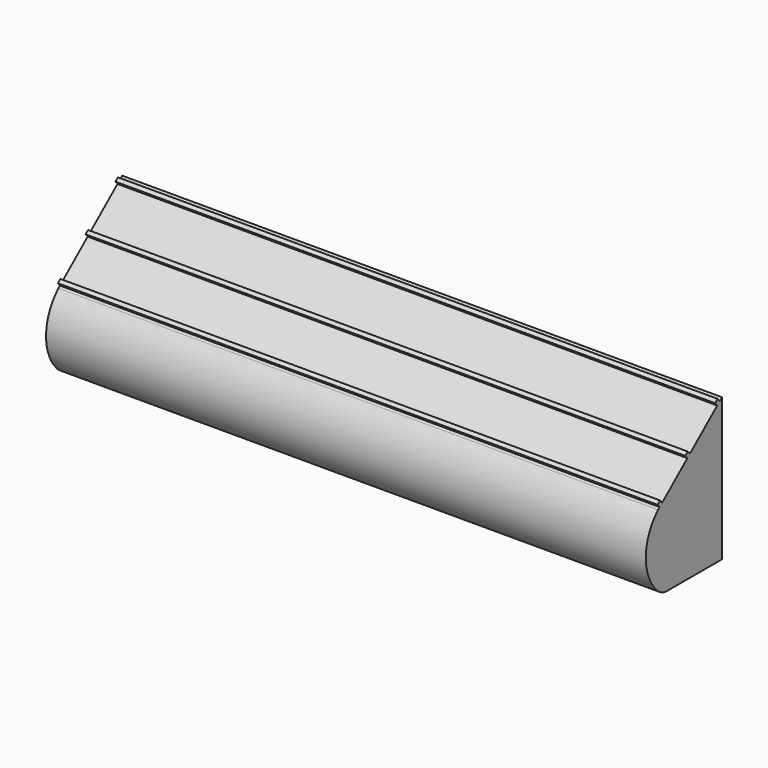
from build123d import *

# Parameters (mm, degrees)
F1_DEPTH    = 55.5
F2_DEPTH    = 297.5
F3_T        = 4
F3_T3_DEPTH = 305.5
F4_R        = 9
F5_R        = 9


# Not quite as in the source:
# - a shell that OpenCascade refuses in one call is made with other operations: the cavity is built on its own and cut out
# - a feature names something its author has since deleted; it is built from what else it names


with BuildPart() as f1:
    # F0 (on Right) → F1 (new body)
    with BuildSketch(Plane.YZ):
        with BuildLine():
            Line((-572.7275457045, -8.2819332473), (-535.7275457045, -8.2819332473))
            Line((-535.7275457045, -8.2819332473), (-535.7275457045, 62.5302098664))
            Line((-535.7275457045, 62.5302098664), (-537.1212494235, 61.363881769))
            Line((-537.1212494235, 61.363881769), (-538.6550321213, 60.0803278606))
            Line((-538.6550321213, 60.0803278606), (-555.619452014, 45.8835661626))
            Line((-555.619452014, 45.8835661626), (-557.1532347119, 44.6000122542))
            Line((-557.1532347119, 44.6000122542), (-572.8000965488, 31.5058557652))
            Line((-572.8000965488, 31.5058557652), (-574.3338792466, 30.2223018568))
            Line((-574.3338792466, 30.2223018568), (-575.2947741996, 29.4181719927))
            ThreePointArc((-575.2947741996, 29.4181719927), (-582.8883712939, 9.9636162879), (-572.7275457045, -8.2819332473))
        make_face()
        Polygon((-538.6550321213, 60.0803278606), (-537.1212494235, 61.363881769), (-538.404803332, 62.8976644668), (-539.9385860298, 61.6141105584), align=None)
        Polygon((-575.6174331551, 31.7560845546), (-574.3338792466, 30.2223018568), (-572.8000965488, 31.5058557652), (-574.0836504573, 33.0396384631), align=None)
        Polygon((-557.1532347119, 44.6000122542), (-555.619452014, 45.8835661626), (-556.9030059225, 47.4173488605), (-558.4367886203, 46.133794952), align=None)
    extrude(amount=F1_DEPTH)

    # F0 (on Right) → F2 (join)
    with BuildSketch(Plane.YZ):
        with BuildLine():
            Line((-572.7275457045, -8.2819332473), (-535.7275457045, -8.2819332473))
            Line((-535.7275457045, -8.2819332473), (-535.7275457045, 62.5302098664))
            Line((-535.7275457045, 62.5302098664), (-537.1212494235, 61.363881769))
            Line((-537.1212494235, 61.363881769), (-538.6550321213, 60.0803278606))
            Line((-538.6550321213, 60.0803278606), (-555.619452014, 45.8835661626))
            Line((-555.619452014, 45.8835661626), (-557.1532347119, 44.6000122542))
            Line((-557.1532347119, 44.6000122542), (-572.8000965488, 31.5058557652))
            Line((-572.8000965488, 31.5058557652), (-574.3338792466, 30.2223018568))
            Line((-574.3338792466, 30.2223018568), (-575.2947741996, 29.4181719927))
            ThreePointArc((-575.2947741996, 29.4181719927), (-582.8883712939, 9.9636162879), (-572.7275457045, -8.2819332473))
        make_face()
        Polygon((-538.6550321213, 60.0803278606), (-537.1212494235, 61.363881769), (-538.404803332, 62.8976644668), (-539.9385860298, 61.6141105584), align=None)
        Polygon((-575.6174331551, 31.7560845546), (-574.3338792466, 30.2223018568), (-572.8000965488, 31.5058557652), (-574.0836504573, 33.0396384631), align=None)
        Polygon((-557.1532347119, 44.6000122542), (-555.619452014, 45.8835661626), (-556.9030059225, 47.4173488605), (-558.4367886203, 46.133794952), align=None)
    extrude(amount=F2_DEPTH)

    # F3: shell of thickness 4, made by hand


with BuildPart() as f3_core1:
    # F3_t2: copy of F1
    add(f1.part)

    # the walls: a layer under each face that stays
    f3_faces = [f3_core1.faces().sort_by_distance(p)[0] for p in [
        (148.75, -582.8883712939, 9.9636162879),
        (0, -559.3362720247, 27.3078656098),
        (148.75, -574.9756562009, 30.9891932057),
        (148.75, -574.8505418062, 32.3978615088),
        (148.75, -573.441873503, 32.2727471141),
        (148.75, -564.9766656303, 38.0529340097),
        (148.75, -557.7950116661, 45.3669036031),
        (148.75, -557.6698972714, 46.7755719063),
        (148.75, -556.2612289683, 46.6504575116),
        (148.75, -547.1372420677, 52.9819470116),
        (148.75, -539.2968090756, 60.8472192095),
        (148.75, -539.1716946809, 62.2558875126),
        (148.75, -537.7630263777, 62.1307731179),
        (148.75, -536.424397564, 61.9470458177),
        (148.75, -554.2275457045, -8.2819332473),
        (297.5, -559.3362720247, 27.3078656098),
        (148.75, -574.8143267231, 29.8202369247),
    ]]
    thicken(f3_faces, amount=-F3_T, mode=Mode.SUBTRACT)

    # F3_s4 → F3_t3 (cut)
    with BuildSketch(Plane.YZ.offset(-4)):
        Polygon((-574.3902259788, 30.2273064326), (-571.266313851, 32.7894096737), (-568.6992060341, 29.721844278), (-571.7667714298, 27.1547364611), align=None)
        Polygon((-572.795091973, 31.5622024973), (-575.8676619445, 28.9387479484), (-573.3005541276, 25.8711825527), (-570.232988732, 28.4382903696), align=None)
        Polygon((-557.209581444, 44.60501683), (-554.586126895, 41.5324468586), (-551.5185614994, 44.0995546754), (-554.0856693162, 47.1671200711), align=None)
        Polygon((-555.6144474383, 45.9399128948), (-558.6870174097, 43.3164583458), (-556.1199095928, 40.2488929501), (-553.0523441972, 42.816000767), align=None)
        Polygon((-538.7113788535, 60.0853324364), (-536.0879243045, 57.0127624649), (-533.0203589088, 59.5798702818), (-535.5874667257, 62.6474356775), align=None)
        Polygon((-537.1162448477, 61.4202285011), (-540.1888148192, 58.7967739522), (-537.6217070023, 55.7292085565), (-534.5541416067, 58.2963163734), align=None)
    extrude(amount=F3_T3_DEPTH, mode=Mode.SUBTRACT)


with BuildPart() as f1_1:
    add(f1.part)

    # what is left inside the walls is the cavity
    f3_cavity = [f3_core1.part.solids().sort_by_distance(p)[0] for p in [
        (197, -535.767546, 26.516207),
    ]]
    add(f3_cavity, mode=Mode.SUBTRACT)

    # F4
    f4_edges = [f1_1.edges().sort_by_distance(p)[0] for p in [
        (148.75, -572.727546, -8.281933),
    ]]
    fillet(f4_edges, radius=F4_R)

    # F5
    f5_edges = [f1_1.edges().sort_by_distance(p)[0] for p in [
        (148.75, -571.376781, -4.281933),
    ]]
    fillet(f5_edges, radius=F5_R)


solid = f1_1.part
